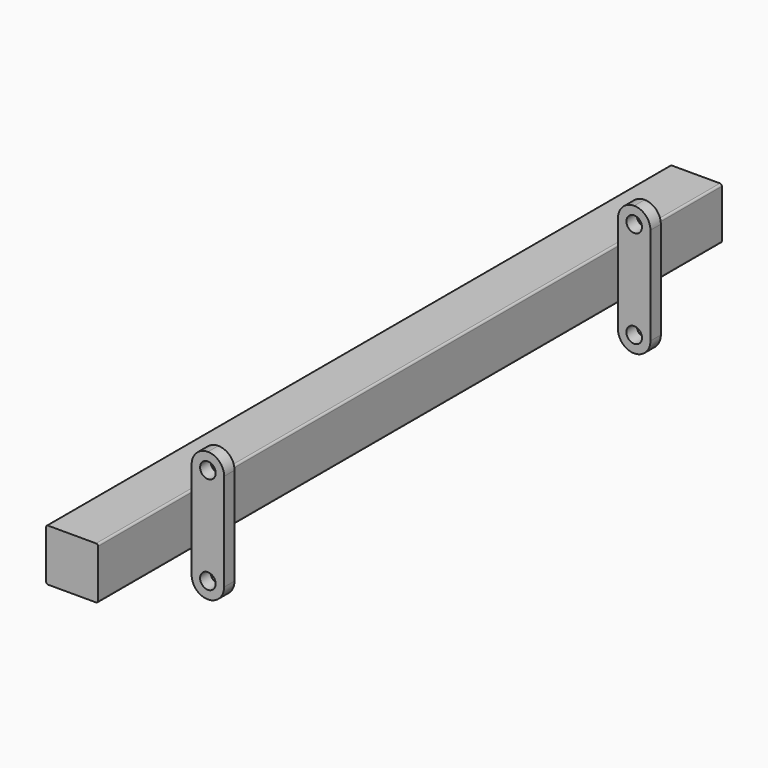
from build123d import *

# Parameters (mm, degrees)
F0_W     = 40
F0_H     = 40
F1_DEPTH = 600
F2_R     = 1.5
F3_W     = 10
F3_H     = 100
F4_DEPTH = 25
F5_R     = 12.49999
F7_D     = 12
F7_DEPTH = 450
F7_TIP   = 3.6051637142


# Not quite as in the source:
# - a fillet or chamfer is up to 0.001 mm smaller than in the source, because OpenCascade refuses the exact size


with BuildPart() as f1:
    # F0 (on Front) → F1 (new body)
    with BuildSketch(Plane.XZ):
        Rectangle(F0_W, F0_H)
    extrude(amount=F1_DEPTH)

    # F2
    f2_edges = [f1.edges().sort_by_distance(p)[0] for p in [
        (-20, -300, 20),
        (-20, -300, -20),
        (20, -300, 20),
        (20, -300, -20),
    ]]
    fillet(f2_edges, radius=F2_R)

    # F3 (on face) → F4 (join)
    with BuildSketch(Plane.YZ.offset(20)):
        with Locations((-505, 0)):
            Rectangle(F3_W, F3_H)
        with Locations((-95, 0)):
            Rectangle(F3_W, F3_H)
    extrude(amount=F4_DEPTH)

    # F5 (radius 12.5 in the source; OpenCascade refuses exactly that, so slightly less here)
    f5_edges = [f1.edges().sort_by_distance(p)[0] for p in [
        (45, -505, 50),
        (20, -505, 50),
        (45, -95, 50),
        (20, -95, 50),
        (45, -95, -50),
        (45, -505, -50),
        (20, -505, -50),
        (20, -95, -50),
    ]]
    fillet(f5_edges, radius=F5_R)

    # F7
    with Locations(Plane.XZ.offset(510)):
        with Locations((32.5, 37.5), (32.5, -37.5)):
            Hole(F7_D / 2, depth=F7_DEPTH)
            with Locations((0, 0, -(F7_DEPTH + F7_TIP / 2))):  # 118° drill point
                Cone(0, F7_D / 2, F7_TIP, mode=Mode.SUBTRACT)


solid = f1.part
